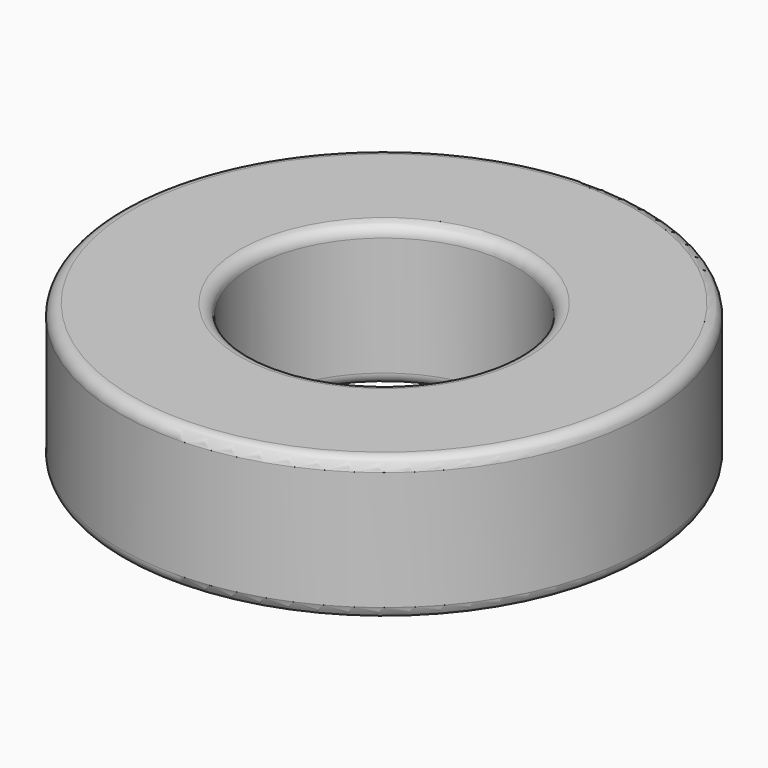
from build123d import *

# Parameters (mm, degrees)
F0_R     = 5.5565
F1_DEPTH = 3
F2_D     = 5.588
F3_R     = 0.25


with BuildPart() as f1:
    # F0 (on Top) → F1 (new body)
    with BuildSketch(Plane.XY):
        Circle(F0_R)
    extrude(amount=F1_DEPTH)

    # F2 (through all)
    with Locations(Plane(origin=(0, 0, 0), x_dir=(1, 0, 0), z_dir=(0, 0, -1))):
        with Locations((0, 0)):
            Hole(F2_D / 2)

    # F3
    f3_edges = [f1.edges().sort_by_distance(p)[0] for p in [
        (-5.5565, 0, 0),
        (-5.5565, 0, 3),
        (-2.794, 0, 3),
        (-2.794, 0, 0),
    ]]
    fillet(f3_edges, radius=F3_R)


solid = f1.part
